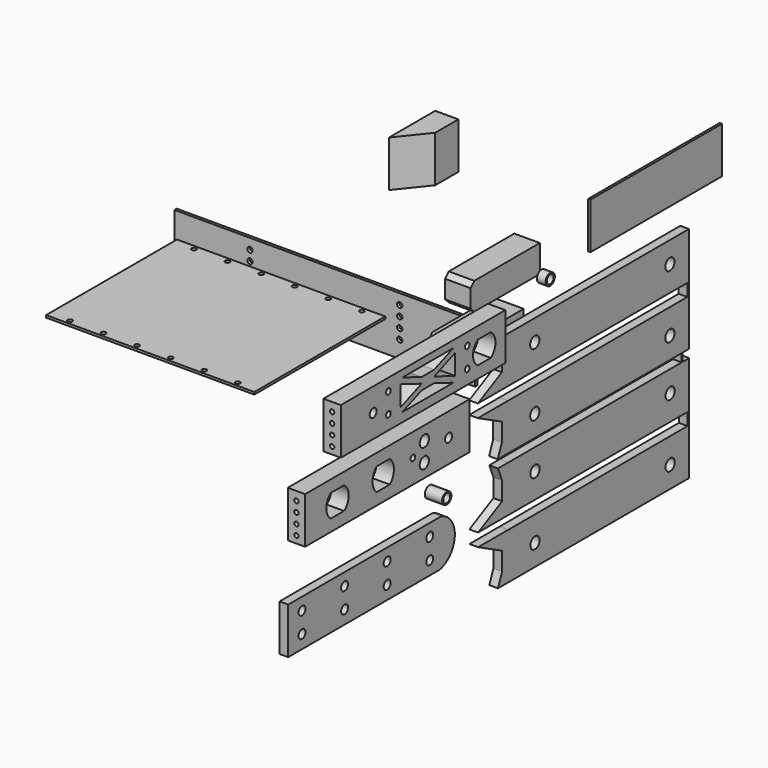
from build123d import *

# Parameters (mm, degrees)
F0_R      = 4.7625
F1_DEPTH  = 19.05
F2_R      = 6.35
F2_R_2    = 4.7625
F3_DEPTH  = 9.525
F4_R      = 6.35
F5_DEPTH  = 9.525
F6_R      = 4.7625
F7_DEPTH  = 19.05
F8_W      = 28
F8_H      = 30
F9_DEPTH  = 95
F10_SIZE  = 5.08
F11_R     = 6.35
F11_R_2   = 4.7625
F12_DEPTH = 19.05
F13_W     = 330.2
F13_H     = 63.5
F14_DEPTH = 3.175
F15_R     = 2.413
F16_DEPTH = 19.05
F17_R     = 2.413
F18_DEPTH = 19.05
F19_R     = 2.9180185013
F20_DEPTH = 3.175
F21_W     = 228.6
F21_H     = 179.67452
F22_DEPTH = 2.54
F23_W     = 34
F23_H     = 16
F24_DEPTH = 85
F25_R     = 3.81
F26_W     = 25
F26_H     = 11
F27_DEPTH = 50
F28_R     = 1.905
F29_R     = 2.54
F30_R     = 6.35
F30_R_2   = 3.175
F31_DEPTH = 19.051
F32_R     = 3.175
F33_DEPTH = 19.051
F34_W     = 180.34
F34_H     = 50.8
F35_DEPTH = 2.54
F37_DEPTH = 50.8
F38_R     = 4.7625
F39_DEPTH = 9.525
F40_R     = 2.54
F41_DEPTH = 221.6923379794


# Not quite as in the source:
# - a feature names something its author has since deleted; it is built from what else it names


with BuildPart() as f1:
    # F0 (on Right) → F1 (new body)
    with BuildSketch(Plane.YZ):
        Polygon((-332.2147077466, 2.7124105329), (-106.4393089773, 2.4784408054), (-106.4393089773, 53.6406252215), (-332.2147077466, 53.6096477747), align=None)
        with Locations((-287.7648304939, 27.9925726354)):
            Circle(F0_R, mode=Mode.SUBTRACT)
        with BuildLine():
            Line((-126.3478304939, 15.5465726354), (-135.3648304939, 15.5465726354))
            Line((-135.3648304939, 15.5465726354), (-144.3818304939, 15.5465726354))
            ThreePointArc((-144.3818304939, 15.5465726354), (-150.7685076522, 27.9925726354), (-144.3818304939, 40.4385726354))
            Line((-144.3818304939, 40.4385726354), (-126.3478304939, 40.4385726354))
            ThreePointArc((-126.3478304939, 40.4385726354), (-119.9611533356, 27.9925726354), (-126.3478304939, 15.5465726354))
        make_face(mode=Mode.SUBTRACT)
    extrude(amount=F1_DEPTH)

    # F17 (on face) → F18 (cut)
    with BuildSketch(Plane.XZ.offset(332.2147077466)):
        with BuildLine():
            ThreePointArc((9.525, 46.4510387747), (7.818751337, 42.3317901117), (11.938, 44.0380387747))
            ThreePointArc((11.938, 44.0380387747), (11.231248663, 45.7442874377), (9.525, 46.4510387747))
        make_face()
        with Locations((9.525, 32.8620387747)):
            Circle(F17_R)
        with Locations((9.525, 21.6860387747)):
            Circle(F17_R)
        with Locations((9.525, 10.5100387747)):
            Circle(F17_R)
    extrude(amount=-F18_DEPTH, mode=Mode.SUBTRACT)

    # F32 (on face) → F33 (cut, through all)
    with BuildSketch(Plane(origin=(0, 0, 0), x_dir=(0, -1, 0), z_dir=(-1, 0, 0))):
        Polygon((175.4130546206, 18.0942449807), (204.1231814975, 29.20619739), (175.4130546206, 40.3181497992), (175.4130546206, 29.20619739), align=None)
        Polygon((249.9933961982, 40.3181497992), (221.2832693213, 29.20619739), (249.9933961982, 18.0942449807), (249.9933961982, 29.20619739), align=None)
        Polygon((212.7032254094, 22.7010805696), (204.1231814975, 22.7010805696), (177.7323673261, 12.4867937303), (212.7032254094, 12.4867937303), align=None)
        Polygon((221.2832693213, 22.7010805696), (212.7032254094, 22.7010805696), (212.7032254094, 12.4867937303), (247.6740834927, 12.4867937303), align=None)
        Polygon((212.7032254094, 35.7113142103), (221.2832693213, 35.7113142103), (247.6740834927, 45.9256010496), (212.7032254094, 45.9256010496), align=None)
        Polygon((204.1231814975, 35.7113142103), (212.7032254094, 35.7113142103), (212.7032254094, 45.9256010496), (177.7323673261, 45.9256010496), align=None)
        with Locations((158.5829828137, 40.3181497992)):
            Circle(F32_R)
        with Locations((266.8234680051, 40.3181497992)):
            Circle(F32_R)
        with Locations((158.5829828137, 18.0942449807)):
            Circle(F32_R)
        with Locations((266.8234680051, 18.0942449807)):
            Circle(F32_R)
    extrude(amount=-F33_DEPTH, mode=Mode.SUBTRACT)


with BuildPart() as f3:
    # F2 (on Right) → F3 (new body)
    with BuildSketch(Plane.YZ):
        with Locations((-32.9032354057, 50.414275378)):
            Circle(F2_R)
        with Locations((-32.9032354057, 50.414275378)):
            Circle(F2_R_2, mode=Mode.SUBTRACT)
    extrude(amount=F3_DEPTH)


with BuildPart() as f5:
    # F4 (on Right) → F5 (new body)
    with BuildSketch(Plane.YZ):
        Polygon((157.4620574125, -34.670151101), (157.4620574125, -29.5203078462), (155.232495817, -29.5178673448), (155.2268587516, -34.6677044292), align=None)
        Polygon((155.232495817, -29.5178673448), (157.4620574125, -29.5203078462), (157.4620574125, 21.6363745818), (-90.9440192401, 21.6024030113), (-104.925731799, 21.6024030113), (-99.2401043375, 7.6732855383), (-99.2401043375, -12.4376901768), (-132.216701885, -29.2483969123), (-90.9468061847, -29.2483969123), align=None)
        with Locations((-54.0916884998, -1.802932184)):
            Circle(F4_R, mode=Mode.SUBTRACT)
        with Locations((131.3283115002, -1.802932184)):
            Circle(F4_R, mode=Mode.SUBTRACT)
        Polygon((157.4620574125, -36.3296834714), (157.4620574125, -34.670151101), (155.2268587516, -34.6677044292), (155.2175832291, -43.1415159214), (157.4620574125, -43.1390590966), align=None)
        Polygon((157.4620574125, -43.1390590966), (155.2175832291, -43.1415159214), (-90.9468061847, -43.4109700305), (-132.216701885, -43.4109700305), (-99.2401043375, -60.2216767659), (-99.2401043375, -80.332652481), (-104.925731799, -94.2617699541), (-90.9440192401, -94.2617699541), (147.4848452582, -94.2943770589), (148.8858715673, -94.2945686607), (157.4620574125, -94.2957415245), align=None)
        with Locations((-54.0916884998, -70.8564347588)):
            Circle(F4_R, mode=Mode.SUBTRACT)
        with Locations((131.3283115002, -70.8564347588)):
            Circle(F4_R, mode=Mode.SUBTRACT)
        Polygon((148.8846508814, -103.2204383231), (148.8858715673, -94.2945686607), (147.4848452582, -94.2943770589), (147.4836245198, -103.220629925), align=None)
        Polygon((157.7795471497, -103.219221873), (148.8846508814, -103.2204383231), (147.4836245198, -103.220629925), (-90.6265295029, -103.2531934435), (-104.6082420618, -103.2531934435), (-98.9226146003, -117.1823109166), (-98.9226146003, -137.2932866316), (-131.8992121478, -154.1039933671), (-90.6293164474, -154.1039933671), (155.5499855542, -154.3734637996), (157.7795471497, -154.375904301), align=None)
        with Locations((-53.7741987626, -126.6585286388)):
            Circle(F4_R, mode=Mode.SUBTRACT)
        with Locations((131.6458012374, -126.6585286388)):
            Circle(F4_R, mode=Mode.SUBTRACT)
        Polygon((157.7795471497, -159.5257475559), (157.7795471497, -154.375904301), (155.5499855542, -154.3734637996), (155.5443484888, -159.5233008841), align=None)
        Polygon((157.7795471497, -161.1852799262), (157.7795471497, -159.5257475559), (155.5443484888, -159.5233008841), (155.5350729663, -167.9971123763), (157.7795471497, -167.9946555514), align=None)
        Polygon((157.7795471497, -167.9946555514), (155.5350729663, -167.9971123763), (-90.6293164474, -168.2665664853), (-131.8992121478, -168.2665664853), (-98.9226146003, -185.0772732208), (-98.9226146003, -205.1882489358), (-104.6082420618, -219.1173664089), (-90.6265295029, -219.1173664089), (157.7795471497, -219.1513379794), align=None)
        with Locations((-53.7741987626, -195.7120312136)):
            Circle(F4_R, mode=Mode.SUBTRACT)
        with Locations((131.6458012374, -195.7120312136)):
            Circle(F4_R, mode=Mode.SUBTRACT)
    extrude(amount=F5_DEPTH)


with BuildPart() as f7:
    # F6 (on Right) → F7 (new body)
    with BuildSketch(Plane.YZ):
        Polygon((-381.1699564363, -63.4196239461), (-155.394557667, -63.6535936735), (-155.394557667, -12.4914092575), (-381.1699564363, -12.5688240225), align=None)
        with BuildLine():
            ThreePointArc((-345.7370791836, -50.5214284561), (-352.1237563419, -38.0754284561), (-345.7370791836, -25.6294284561))
            Line((-345.7370791836, -25.6294284561), (-327.7030791836, -25.6294284561))
            ThreePointArc((-327.7030791836, -25.6294284561), (-321.3164020253, -38.0754284561), (-327.7030791836, -50.5214284561))
            Line((-327.7030791836, -50.5214284561), (-336.7200791836, -50.5214284561))
            Line((-336.7200791836, -50.5214284561), (-345.7370791836, -50.5214284561))
        make_face(mode=Mode.SUBTRACT)
        with Locations((-184.3200791836, -38.0725014655)):
            Circle(F6_R, mode=Mode.SUBTRACT)
    extrude(amount=F7_DEPTH)

    # F15 (on face) → F16 (cut)
    with BuildSketch(Plane.XZ.offset(381.1699564363)):
        with Locations((9.525, -22.140443325)):
            Circle(F15_R)
        with Locations((9.525, -33.316443325)):
            Circle(F15_R)
        with Locations((9.525, -44.492443325)):
            Circle(F15_R)
        with Locations((9.525, -55.668443325)):
            Circle(F15_R)
    extrude(amount=-F16_DEPTH, mode=Mode.SUBTRACT)

    # F30 (on face) → F31 (cut, through all)
    with BuildSketch(Plane(origin=(0, 0, 0), x_dir=(0, -1, 0), z_dir=(-1, 0, 0))):
        Polygon((274.0023015713, -50.5214284561), (283.0447015713, -50.5214284561), (283.0447015713, -25.6294284561), (264.9599015713, -25.6294284561), (264.9599015713, -50.5214284561), align=None)
        with BuildLine():
            Line((283.0447015713, -25.6294284561), (283.0447015713, -50.5214284561))
            ThreePointArc((283.0447015713, -50.5214284561), (288.6736622572, -38.0754284561), (283.0447015713, -25.6294284561))
        make_face()
        with BuildLine():
            ThreePointArc((264.9599015713, -25.6294284561), (259.3309408853, -38.0754284561), (264.9599015713, -50.5214284561))
            Line((264.9599015713, -50.5214284561), (264.9599015713, -25.6294284561))
        make_face()
        with Locations((217.5404429436, -27.6374015957)):
            Circle(F30_R)
        with Locations((217.5404429436, -48.6397631466)):
            Circle(F30_R)
        with Locations((233.2088649273, -37.6385264099)):
            Circle(F30_R_2)
    extrude(amount=-F31_DEPTH, mode=Mode.SUBTRACT)


with BuildPart() as f9:
    # F8 (on Front) → F9 (new body)
    with BuildSketch(Plane.XZ):
        with Locations((-42.2337934971, 44.8543777317)):
            Rectangle(F8_W, F8_H)
    extrude(amount=F9_DEPTH)

    # F10
    f10_edges = [f9.edges().sort_by_distance(p)[0] for p in [
        (-42.233793, -95, 59.854378),
        (-42.233793, -95, 29.854378),
    ]]
    chamfer(f10_edges, length=F10_SIZE)


with BuildPart() as f12:
    # F11 (on Right) → F12 (new body)
    with BuildSketch(Plane.YZ):
        with Locations((-186.7705434561, -95.4420268536)):
            Circle(F11_R)
        with Locations((-186.7705434561, -95.4420268536)):
            Circle(F11_R_2, mode=Mode.SUBTRACT)
    extrude(amount=F12_DEPTH)


with BuildPart() as f14:
    # F13 (on Front) → F14 (new body)
    with BuildSketch(Plane.XZ):
        with Locations((-261.6744421959, -68.3120494597)):
            Rectangle(F13_W, F13_H)
    extrude(amount=F14_DEPTH)

    # F19 (on face) → F20 (cut, through all)
    with BuildSketch(Plane.XZ.offset(3.175)):
        with Locations((-343.8294721959, -47.9920494597)):
            Circle(F19_R)
        with Locations((-343.8294721959, -59.1680494597)):
            Circle(F19_R)
        with Locations((-343.8294721959, -70.3440494597)):
            Circle(F19_R)
        with Locations((-343.8294721959, -81.5200494597)):
            Circle(F19_R)
        with Locations((-179.5194121959, -70.3440494597)):
            Circle(F19_R)
        with Locations((-179.5194121959, -59.1680494597)):
            Circle(F19_R)
        with BuildLine():
            Line((-179.5194121959, -47.9920494597), (-182.4374306972, -47.9920494597))
            ThreePointArc((-182.4374306972, -47.9920494597), (-179.5194121959, -50.910067961), (-176.6013936946, -47.9920494597))
            ThreePointArc((-176.6013936946, -47.9920494597), (-177.456061526, -45.9286987898), (-179.5194121959, -45.0740309584))
            Line((-179.5194121959, -45.0740309584), (-179.5194121959, -47.9920494597))
        make_face()
        with Locations((-179.5194121959, -81.5200494597)):
            Circle(F19_R)
        with BuildLine():
            ThreePointArc((-179.5194121959, -45.0740309584), (-181.5827628658, -45.9286987898), (-182.4374306972, -47.9920494597))
            Line((-182.4374306972, -47.9920494597), (-179.5194121959, -47.9920494597))
            Line((-179.5194121959, -47.9920494597), (-179.5194121959, -45.0740309584))
        make_face()
    extrude(amount=-F20_DEPTH, mode=Mode.SUBTRACT)


with BuildPart() as f22:
    # F21 (on Top) → F22 (new body)
    with BuildSketch(Plane.XY):
        with Locations((-229.5971042633, -193.1023826678)):
            Rectangle(F21_W, F21_H)
    extrude(amount=F22_DEPTH)

    # F40 (on face) → F41 (cut, through all)
    with BuildSketch(Plane.XY.offset(2.54)):
        with Locations((-321.3791251183, -108.0276226678)):
            Circle(F40_R)
        with Locations((-284.5491251183, -108.0276226678)):
            Circle(F40_R)
        with Locations((-247.7191251183, -108.0276226678)):
            Circle(F40_R)
        with Locations((-210.8891251183, -108.0276226678)):
            Circle(F40_R)
        with Locations((-174.0591251183, -108.0276226678)):
            Circle(F40_R)
        with Locations((-137.2291251183, -108.0276226678)):
            Circle(F40_R)
        with Locations((-284.5491251183, -278.1771426678)):
            Circle(F40_R)
        with Locations((-321.3791251183, -278.1771426678)):
            Circle(F40_R)
        with Locations((-247.7191251183, -278.1771426678)):
            Circle(F40_R)
        with Locations((-174.0591251183, -278.1771426678)):
            Circle(F40_R)
        with Locations((-137.2291251183, -278.1771426678)):
            Circle(F40_R)
        with Locations((-210.8891251183, -278.1771426678)):
            Circle(F40_R)
    extrude(amount=-F41_DEPTH, mode=Mode.SUBTRACT)


with BuildPart() as f24:
    # F23 (on Front) → F24 (new body)
    with BuildSketch(Plane.XZ):
        with Locations((-62.9992904067, -17.5642086267)):
            Rectangle(F23_W, F23_H)
    extrude(amount=F24_DEPTH)

    # F25
    f25_edges = [f24.edges().sort_by_distance(p)[0] for p in [
        (-62.99929, -85, -25.564209),
        (-62.99929, -85, -9.564209),
    ]]
    fillet(f25_edges, radius=F25_R)


with BuildPart() as f27:
    # F26 (on Front) → F27 (new body)
    with BuildSketch(Plane.XZ):
        with Locations((-84.0954952087, -46.9318069518)):
            Rectangle(F26_W, F26_H)
    extrude(amount=F27_DEPTH)

    # F28
    f28_edges = [f27.edges().sort_by_distance(p)[0] for p in [
        (-84.095495, -50, -41.431807),
        (-96.595495, -50, -46.931807),
        (-84.095495, -50, -52.431807),
        (-71.595495, -50, -46.931807),
    ]]
    fillet(f28_edges, radius=F28_R)

    # F29
    f29_edges = [f27.edges().sort_by_distance(p)[0] for p in [
        (-71.595495, 0, -46.931807),
        (-84.095495, 0, -41.431807),
        (-96.595495, 0, -46.931807),
        (-84.095495, 0, -52.431807),
    ]]
    fillet(f29_edges, radius=F29_R)


with BuildPart() as f35:
    # F34 (on Right) → F35 (new body)
    with BuildSketch(Plane.YZ):
        with Locations((121.262312187, 73.6839345932)):
            Rectangle(F34_W, F34_H)
    extrude(amount=F35_DEPTH)


with BuildPart() as f37:
    # F36 (on Top) → F37 (new body)
    with BuildSketch(Plane.XY):
        Polygon((-262.3816430569, 149.1663137674), (-262.3816430569, 85.6663137674), (-236.9816430569, 117.4163137674), (-236.9816430569, 149.1663137674), align=None)
    extrude(amount=F37_DEPTH)


with BuildPart() as f39:
    # F38 (on Right) → F39 (new body)
    with BuildSketch(Plane.YZ):
        with BuildLine():
            ThreePointArc((-163.8942807913, -144.9705064297), (-163.8182755561, -142.9741592804), (-163.8942807913, -140.9778121311))
            Line((-163.8942807913, -140.9778121311), (-163.8942807913, -144.9705064297))
        make_face()
        with BuildLine():
            Line((-182.5617104769, -117.8159223318), (-392.4942807913, -117.8159223318))
            Line((-392.4942807913, -117.8159223318), (-392.4942807913, -168.6159223318))
            Line((-392.4942807913, -168.6159223318), (-184.4284534454, -168.6159223318))
            ThreePointArc((-184.4284534454, -168.6159223318), (-170.250111038, -160.1898307896), (-163.8942807913, -144.9705064297))
            Line((-163.8942807913, -144.9705064297), (-163.8942807913, -140.9778121311))
            ThreePointArc((-163.8942807913, -140.9778121311), (-169.6312860792, -126.4980829226), (-182.5617104769, -117.8159223318))
        make_face()
        with Locations((-373.5028803349, -153.9315131245)):
            Circle(F38_R, mode=Mode.SUBTRACT)
        with Locations((-315.0828803349, -153.9315131245)):
            Circle(F38_R, mode=Mode.SUBTRACT)
        with Locations((-256.6628803349, -153.9315131245)):
            Circle(F38_R, mode=Mode.SUBTRACT)
        with Locations((-198.2428803349, -153.9315131245)):
            Circle(F38_R, mode=Mode.SUBTRACT)
        with Locations((-373.5028803349, -131.3255131245)):
            Circle(F38_R, mode=Mode.SUBTRACT)
        with Locations((-315.0828803349, -131.3255131245)):
            Circle(F38_R, mode=Mode.SUBTRACT)
        with Locations((-256.6628803349, -131.3255131245)):
            Circle(F38_R, mode=Mode.SUBTRACT)
        with Locations((-198.2428803349, -131.3255131245)):
            Circle(F38_R, mode=Mode.SUBTRACT)
    extrude(amount=F39_DEPTH)


solid = Compound([f1.part, f3.part, f5.part, f7.part, f9.part, f12.part, f14.part, f22.part, f24.part, f27.part, f35.part, f37.part, f39.part])
